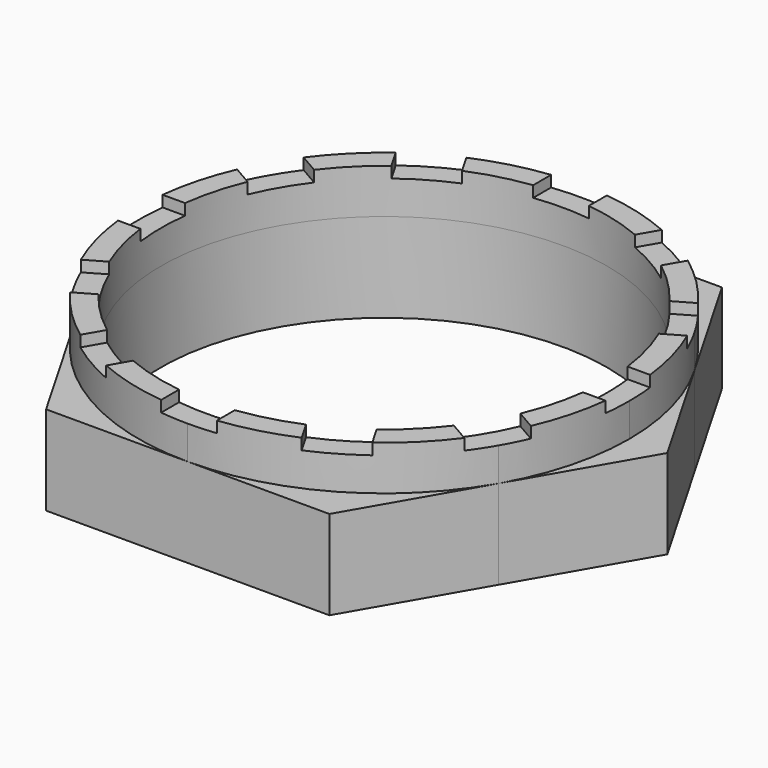
from build123d import *

# Parameters (mm, degrees)
F1_R     = 12.7
F2_DEPTH = 2.54
F3_DEPTH = 5.08
F5_DEPTH = 0.635


with BuildPart() as f2:
    # F1 (on Top) → F2 (new body)
    with BuildSketch(Plane.XY):
        with BuildLine():
            ThreePointArc((12.0983740846, -6.9850013965), (13.4939835846, -3.6157028389), (13.97, 0))
            ThreePointArc((13.97, 0), (13.493983574, 3.6157028785), (12.0983740436, 6.9850014675))
            ThreePointArc((12.0983740436, 6.9850014675), (6.9849992663, 12.0983753145), (0, 13.97))
            ThreePointArc((0, 13.97), (-6.9849993112, 12.0983752885), (-12.0983740955, 6.9850013775))
            ThreePointArc((-12.0983740955, 6.9850013775), (-13.97, 8.2e-08), (-12.0983741776, -6.9850012354))
            ThreePointArc((-12.0983741776, -6.9850012354), (-6.9849993823, -12.0983752475), (0, -13.97))
            ThreePointArc((0, -13.97), (6.9849993017, -12.098375294), (12.0983740846, -6.9850013965))
        make_face()
        Circle(F1_R, mode=Mode.SUBTRACT)
    extrude(amount=F2_DEPTH)

    # F4 (on face) → F5 (cut)
    with BuildSketch(Plane.XY.offset(2.54)):
        with BuildLine():
            Line((-12.6003906189, 1.5875), (-13.8795080514, 1.5875))
            ThreePointArc((-13.8795080514, 1.5875), (-13.97, 0), (-13.8795080514, -1.5875))
            Line((-13.8795080514, -1.5875), (-12.6003906189, -1.5875))
            ThreePointArc((-12.6003906189, -1.5875), (-12.7, 0), (-12.6003906189, 1.5875))
        make_face()
        with BuildLine():
            Line((-10.1185083736, 7.675010638), (-11.2262565646, 8.3145693542))
            ThreePointArc((-11.2262565646, 8.3145693542), (-12.0983748909, 6.985), (-12.8137565646, 5.5649386972))
            Line((-12.8137565646, 5.5649386972), (-11.7060083736, 4.925379981))
            ThreePointArc((-11.7060083736, 4.925379981), (-10.9985226281, 6.35), (-10.1185083736, 7.675010638))
        make_face()
        with BuildLine():
            ThreePointArc((-5.5649386972, 12.8137565646), (-6.985, 12.0983748909), (-8.3145693542, 11.2262565646))
            Line((-8.3145693542, 11.2262565646), (-7.675010638, 10.1185083736))
            ThreePointArc((-7.675010638, 10.1185083736), (-6.35, 10.9985226281), (-4.925379981, 11.7060083736))
            Line((-4.925379981, 11.7060083736), (-5.5649386972, 12.8137565646))
        make_face()
        with BuildLine():
            ThreePointArc((1.5875, 13.8795080514), (0, 13.97), (-1.5875, 13.8795080514))
            Line((-1.5875, 13.8795080514), (-1.5875, 12.6003906189))
            ThreePointArc((-1.5875, 12.6003906189), (0, 12.7), (1.5875, 12.6003906189))
            Line((1.5875, 12.6003906189), (1.5875, 13.8795080514))
        make_face()
        with BuildLine():
            ThreePointArc((8.3145693542, 11.2262565646), (6.985, 12.0983748909), (5.5649386972, 12.8137565646))
            Line((5.5649386972, 12.8137565646), (4.925379981, 11.7060083736))
            ThreePointArc((4.925379981, 11.7060083736), (6.35, 10.9985226281), (7.675010638, 10.1185083736))
            Line((7.675010638, 10.1185083736), (8.3145693542, 11.2262565646))
        make_face()
        with BuildLine():
            ThreePointArc((13.97, 0), (13.9473586653, 0.7950385278), (13.8795080514, 1.5875))
            Line((13.8795080514, 1.5875), (12.6003906189, 1.5875))
            ThreePointArc((12.6003906189, 1.5875), (12.6750731923, 0.7953109893), (12.7, 0))
            ThreePointArc((12.7, 0), (12.6750731923, -0.7953109893), (12.6003906189, -1.5875))
            Line((12.6003906189, -1.5875), (13.8795080514, -1.5875))
            ThreePointArc((13.8795080514, -1.5875), (13.9473586653, -0.7950385278), (13.97, 0))
        make_face()
        with BuildLine():
            ThreePointArc((11.2262565646, -8.3145693542), (12.0983748909, -6.985), (12.8137565646, -5.5649386972))
            Line((12.8137565646, -5.5649386972), (11.7060083736, -4.925379981))
            ThreePointArc((11.7060083736, -4.925379981), (10.9985226281, -6.35), (10.1185083736, -7.675010638))
            Line((10.1185083736, -7.675010638), (11.2262565646, -8.3145693542))
        make_face()
        with BuildLine():
            Line((4.925379981, -11.7060083736), (5.5649386972, -12.8137565646))
            ThreePointArc((5.5649386972, -12.8137565646), (6.985, -12.0983748909), (8.3145693542, -11.2262565646))
            Line((8.3145693542, -11.2262565646), (7.675010638, -10.1185083736))
            ThreePointArc((7.675010638, -10.1185083736), (6.35, -10.9985226281), (4.925379981, -11.7060083736))
        make_face()
        with BuildLine():
            Line((-1.5875, -12.6003906189), (-1.5875, -13.8795080514))
            ThreePointArc((-1.5875, -13.8795080514), (0, -13.97), (1.5875, -13.8795080514))
            Line((1.5875, -13.8795080514), (1.5875, -12.6003906189))
            ThreePointArc((1.5875, -12.6003906189), (0, -12.7), (-1.5875, -12.6003906189))
        make_face()
        with BuildLine():
            Line((-7.675010638, -10.1185083736), (-8.3145693542, -11.2262565646))
            ThreePointArc((-8.3145693542, -11.2262565646), (-6.985, -12.0983748909), (-5.5649386972, -12.8137565646))
            Line((-5.5649386972, -12.8137565646), (-4.925379981, -11.7060083736))
            ThreePointArc((-4.925379981, -11.7060083736), (-6.35, -10.9985226281), (-7.675010638, -10.1185083736))
        make_face()
        with BuildLine():
            Line((-11.7060083736, -4.925379981), (-12.8137565646, -5.5649386972))
            ThreePointArc((-12.8137565646, -5.5649386972), (-12.0983748909, -6.985), (-11.2262565646, -8.3145693542))
            Line((-11.2262565646, -8.3145693542), (-10.1185083736, -7.675010638))
            ThreePointArc((-10.1185083736, -7.675010638), (-10.9985226281, -6.35), (-11.7060083736, -4.925379981))
        make_face()
        with BuildLine():
            ThreePointArc((12.8137565646, 5.5649386972), (12.0983748909, 6.985), (11.2262565646, 8.3145693542))
            Line((11.2262565646, 8.3145693542), (10.1185083736, 7.675010638))
            ThreePointArc((10.1185083736, 7.675010638), (10.9985226281, 6.35), (11.7060083736, 4.925379981))
            Line((11.7060083736, 4.925379981), (12.8137565646, 5.5649386972))
        make_face()
    extrude(amount=-F5_DEPTH, mode=Mode.SUBTRACT)


with BuildPart() as f3:
    # F1 (on Top) → F3 (new body)
    with BuildSketch(Plane.XY):
        with BuildLine():
            ThreePointArc((-12.0983740955, 6.9850013775), (-6.9849993112, 12.0983752885), (0, 13.97))
            Line((0, 13.97), (-8.0655832606, 13.97))
            Line((-8.0655832606, 13.97), (-12.0983740955, 6.9850013775))
        make_face()
        with BuildLine():
            ThreePointArc((-12.0983741776, -6.9850012354), (-13.97, 8.2e-08), (-12.0983740955, 6.9850013775))
            Line((-12.0983740955, 6.9850013775), (-16.1311665212, 0))
            Line((-16.1311665212, 0), (-12.0983741776, -6.9850012354))
        make_face()
        with BuildLine():
            Line((-8.0655832606, -13.97), (0, -13.97))
            ThreePointArc((0, -13.97), (-6.9849993823, -12.0983752475), (-12.0983741776, -6.9850012354))
            Line((-12.0983741776, -6.9850012354), (-8.0655832606, -13.97))
        make_face()
        with BuildLine():
            Line((8.0655832606, -13.97), (12.0983740846, -6.9850013965))
            ThreePointArc((12.0983740846, -6.9850013965), (6.9849993017, -12.098375294), (0, -13.97))
            Line((0, -13.97), (8.0655832606, -13.97))
        make_face()
        with BuildLine():
            ThreePointArc((12.0983740436, 6.9850014675), (13.493983574, 3.6157028785), (13.97, 0))
            ThreePointArc((13.97, 0), (13.4939835846, -3.6157028389), (12.0983740846, -6.9850013965))
            Line((12.0983740846, -6.9850013965), (16.1311665212, 0))
            Line((16.1311665212, 0), (12.0983740436, 6.9850014675))
        make_face()
        with BuildLine():
            ThreePointArc((0, 13.97), (6.9849992663, 12.0983753145), (12.0983740436, 6.9850014675))
            Line((12.0983740436, 6.9850014675), (8.0655832606, 13.97))
            Line((8.0655832606, 13.97), (0, 13.97))
        make_face()
        with BuildLine():
            ThreePointArc((12.0983740846, -6.9850013965), (13.4939835846, -3.6157028389), (13.97, 0))
            ThreePointArc((13.97, 0), (13.493983574, 3.6157028785), (12.0983740436, 6.9850014675))
            ThreePointArc((12.0983740436, 6.9850014675), (6.9849992663, 12.0983753145), (0, 13.97))
            ThreePointArc((0, 13.97), (-6.9849993112, 12.0983752885), (-12.0983740955, 6.9850013775))
            ThreePointArc((-12.0983740955, 6.9850013775), (-13.97, 8.2e-08), (-12.0983741776, -6.9850012354))
            ThreePointArc((-12.0983741776, -6.9850012354), (-6.9849993823, -12.0983752475), (0, -13.97))
            ThreePointArc((0, -13.97), (6.9849993017, -12.098375294), (12.0983740846, -6.9850013965))
        make_face()
        Circle(F1_R, mode=Mode.SUBTRACT)
    extrude(amount=-F3_DEPTH)


solid = Compound([f2.part, f3.part])
